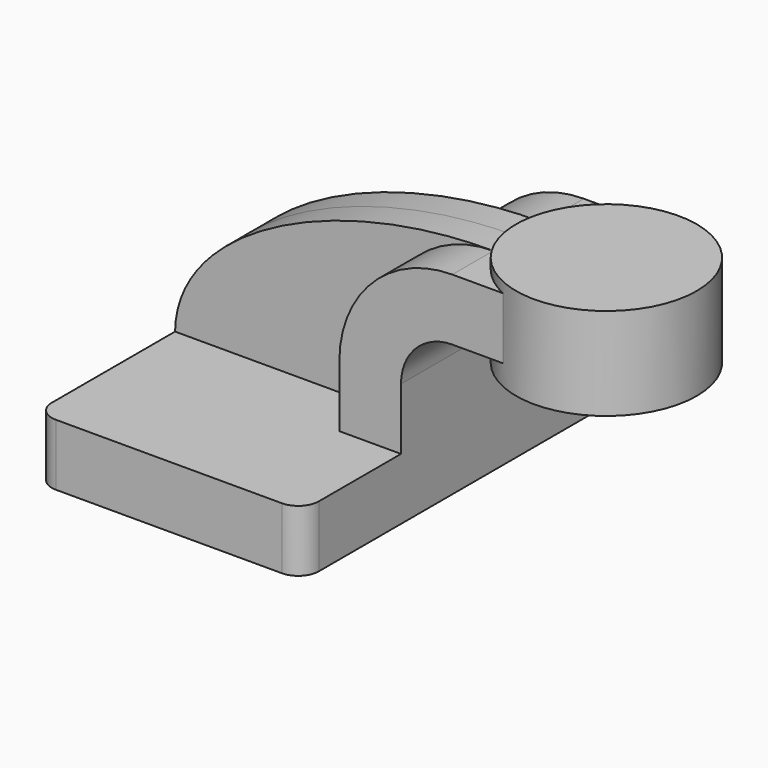
from build123d import *

# Parameters (mm, degrees)
F1_DEPTH = 63.5
F0_W     = 22.86
F0_H     = 19.05
F2_DEPTH = 25.4
F3_DEPTH = 9.525
F5_R     = 6.35


with BuildPart() as f1:
    # F0 (on Front) → F1 (new body, symmetric)
    with BuildSketch(Plane.XZ):
        Polygon((-41.275, 9.525), (-41.275, -9.525), (41.275, -9.525), (41.275, 9.525), (22.225, 9.525), align=None)
    extrude(amount=F1_DEPTH, both=True)

    # F0 (on Front) → F2 (join, symmetric)
    with BuildSketch(Plane.XZ):
        with BuildLine():
            Line((22.225, 9.525), (41.275, 9.525))
            Line((41.275, 9.525), (41.275, 28.575))
            ThreePointArc((41.275, 28.575), (45.9246798487, 39.8003201513), (57.15, 44.45))
            Line((57.15, 44.45), (61.595, 44.45))
            Line((61.595, 44.45), (61.595, 63.5))
            Line((61.595, 63.5), (57.15, 63.5))
            ThreePointArc((57.15, 63.5), (32.4542956671, 53.2707043329), (22.225, 28.575))
            Line((22.225, 28.575), (22.225, 9.525))
        make_face()
        with Locations((73.025, 53.975)):
            Rectangle(F0_W, F0_H)
    extrude(amount=F2_DEPTH, both=True)

    # F0 (on Front) → F3 (join, symmetric)
    with BuildSketch(Plane.XZ):
        with BuildLine():
            add(Edge.make_bspline(
                [(-41.275, 9.525), (-40.8756434917, 39.7976487875), (7.9142833129, 63.7873858213), (57.15, 63.5)],
                knots=[0, 0, 0, 0, 112.2532015134, 112.2532015134, 112.2532015134, 112.2532015134], degree=3))
            Line((-41.275, 9.525), (22.225, 9.525))
            Line((22.225, 9.525), (22.225, 28.575))
            ThreePointArc((22.225, 28.575), (32.4542956671, 53.2707043329), (57.15, 63.5))
        make_face()
    extrude(amount=F3_DEPTH, both=True)

    # F0 (on Front) → F4 (revolve)
    with BuildSketch(Plane.XZ):
        Polygon((84.455, 66.675), (84.455, 63.5), (84.455, 44.45), (84.455, 38.1), (112.395, 38.1), (112.395, 66.675), align=None)
    revolve(axis=Axis((84.455, 0, 52.3875), (0, 0, 1)))

    # F5
    f5_edges = [f1.edges().sort_by_distance(p)[0] for p in [
        (-41.275, -63.5, 0),
        (41.275, -63.5, 0),
        (41.275, 63.5, 0),
        (-41.275, 63.5, 0),
    ]]
    fillet(f5_edges, radius=F5_R)


solid = f1.part
